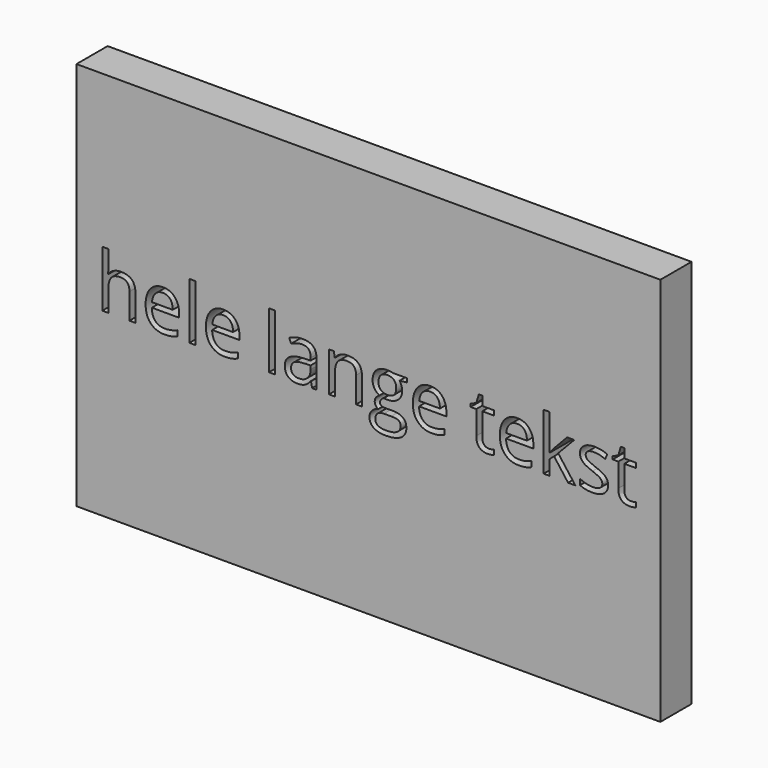
from build123d import *

# Parameters (mm, degrees)
F0_W         = 150
F0_H         = 100
F1_DEPTH     = 10
F2_TEXT_SIZE = 19.0395240119
F3_DEPTH     = 10.001


# Not quite as in the source:
# - Text() gives the source's letters only with a copy of the font that has no kerning and outlines rounded to 1/6400 em; it was checked with that copy


with BuildPart() as f1:
    # F0 (on Front) → F1 (new body)
    with BuildSketch(Plane.XZ):
        Rectangle(F0_W, F0_H)
    extrude(amount=F1_DEPTH)

    # F2 (on face) → F3 (cut, through all)
    with BuildSketch(Plane.XZ.offset(10)):
        with Locations((-70, -3.6153539518)):
            Text('hele lange tekst', F2_TEXT_SIZE, font='Open Sans', text_align=(TextAlign.LEFT, TextAlign.BOTTOM))
    extrude(amount=-F3_DEPTH, mode=Mode.SUBTRACT)


solid = f1.part
